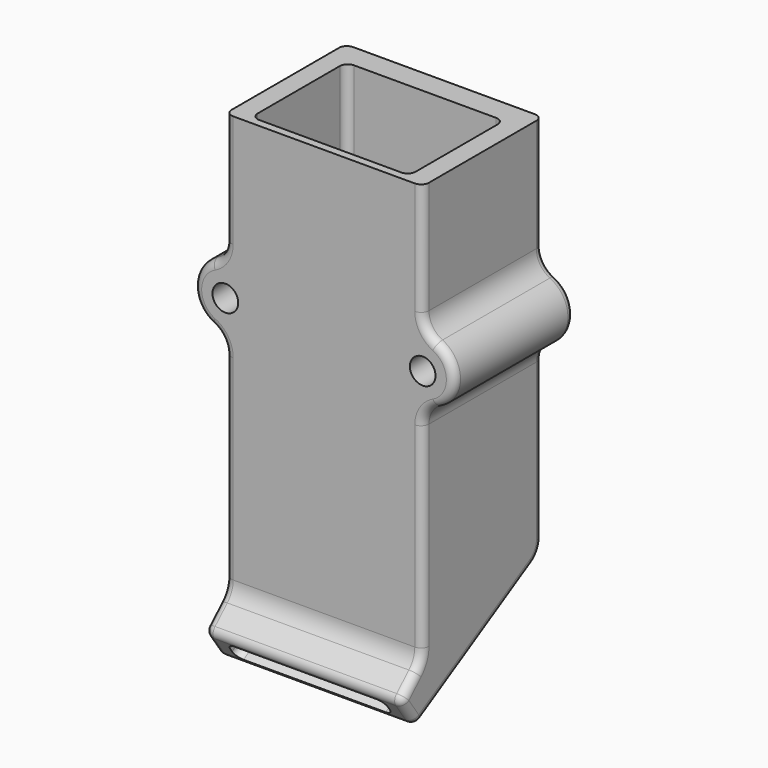
from build123d import *

# Parameters (mm, degrees)
F1_DEPTH = 12.5
F3_DEPTH = 10
F4_R     = 4
F5_DEPTH = 19
F6_R     = 1.625
F7_DEPTH = 19
F8_R     = 3
F9_R     = 1


with BuildPart() as f1:
    # F0 (on Right) → F1 (new body, symmetric)
    with BuildSketch(Plane.YZ):
        Polygon((10.5, -48.5), (10.5, 0.0014402197), (-8.5, 0.0014402197), (-8.5, -52.9983094265), (-11.9987755675, -56.3131838999), (-9.418584287, -60), align=None)
    extrude(amount=F1_DEPTH, both=True)

    # F2 (on Right) → F3 (cut, symmetric)
    with BuildSketch(Plane.YZ):
        Polygon((7.5, 0.0014402197), (-7.5, 0.0014402197), (-7.5, -53.428419387), (-11.4190800593, -57.1415064933), (-9.9941380171, -59.1775955626), (7.5, -49.0773502692), align=None)
    extrude(amount=F3_DEPTH, both=True, mode=Mode.SUBTRACT)

    # F4 (on face) → F5 (join, through all)
    with BuildSketch(Plane.XZ.offset(8.5)):
        with Locations((12.5, -20.5985597803)):
            Circle(F4_R)
        with Locations((-12.5, -20.5985597803)):
            Circle(F4_R)
    extrude(amount=-F5_DEPTH)

    # F6 (on face) → F7 (cut, through all)
    with BuildSketch(Plane.XZ.offset(8.5)):
        with Locations((-12.5, -20.5985597803)):
            Circle(F6_R)
        with Locations((12.5, -20.5985597803)):
            Circle(F6_R)
    extrude(amount=-F7_DEPTH, mode=Mode.SUBTRACT)

    # F8
    f8_edges = [f1.edges().sort_by_distance(p)[0] for p in [
        (-12.5, 1, -16.59856),
        (-12.5, 1, -24.59856),
        (12.5, 1, -16.59856),
        (12.5, 1, -24.59856),
        (-10, 0, -17.476061),
        (-10, 0, -23.721059),
        (10, 0, -17.476061),
        (10, 0, -23.721059),
        (0, 7.5, -49.07735),
        (0, -8.5, -52.998309),
        (0, 10.5, -48.5),
    ]]
    fillet(f8_edges, radius=F8_R)

    # F9
    f9_edges = [f1.edges().sort_by_distance(p)[0] for p in [
        (10, -7.5, -8.133496),
        (-10, -7.5, -8.133496),
        (10, 7.5, -8.133496),
        (-10, 7.5, -8.133496),
        (-10, -1.997069, -54.560486),
        (10, -1.997069, -54.560486),
        (10, -9.45954, -55.284963),
        (-10, -9.45954, -55.284963),
        (0, -7.5, -53.428419),
        (-12.5, -8.5, -39.315547),
        (-16.5, -8.5, -20.59856),
        (-12.5, -8.5, -7.136282),
        (-12.5, -10.70868, -58.156592),
        (-12.5, -0.209292, -54.683013),
        (-12.5, 10.5, -36.845532),
        (12.5, 10.5, -36.845532),
        (0, 9, -49.366025),
        (12.5, -8.5, -39.315547),
        (16.5, -8.5, -20.59856),
        (12.5, -0.209292, -54.683013),
        (0, -11.998776, -56.313184),
        (12.5, -10.70868, -58.156592),
        (0, -9.418584, -60),
    ]]
    fillet(f9_edges, radius=F9_R)


solid = f1.part
